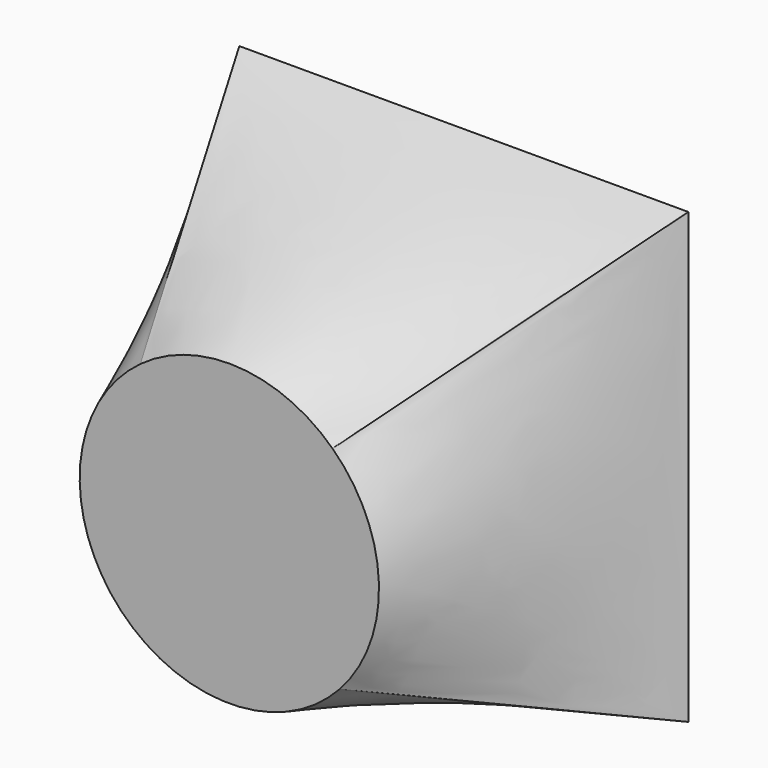
from build123d import *

# Parameters (mm, degrees)
F0_W = 228.6
F0_H = 228.6


with BuildPart() as f3:
    # F0 (on Front) → F3 section 0
    with BuildSketch(Plane.XZ):
        Rectangle(F0_W, F0_H)
    # F2 (on offset) → F3 section 1
    with BuildSketch(Plane.XZ.offset(101.6)):
        with BuildLine():
            ThreePointArc((14.446943, 17.083864), (-33.349733, 37.951791), (-83.371643, 23.193705))
            ThreePointArc((-83.371643, 23.193705), (-114.013509, -31.498553), (-93.272294, -90.65909))
            ThreePointArc((-93.272294, -90.65909), (-37.386199, -114.296657), (18.047259, -89.616263))
            ThreePointArc((18.047259, -89.616263), (38.056658, -35.530293), (14.446943, 17.083864))
        make_face()
    loft()


solid = f3.part
